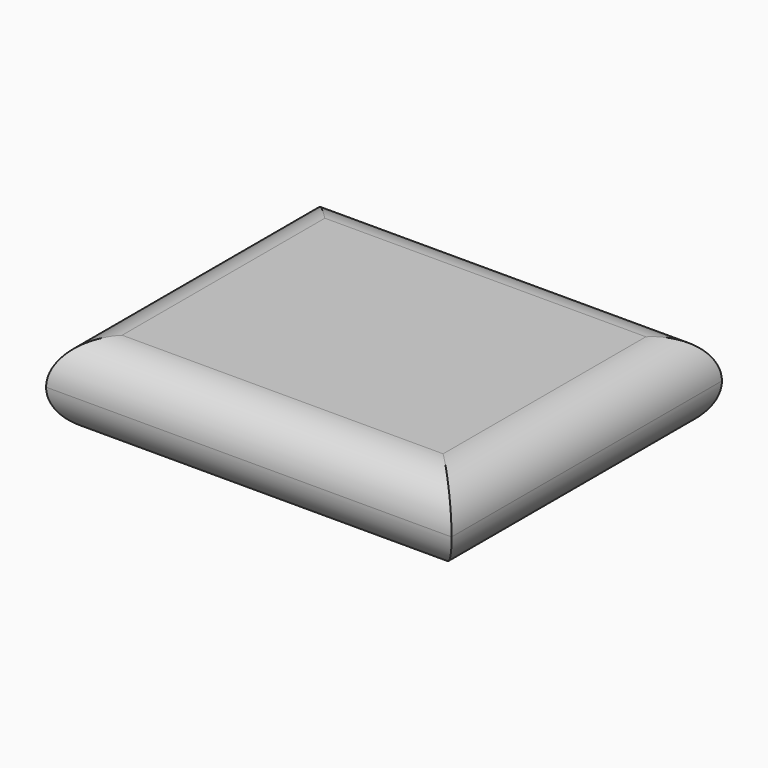
from build123d import *

# Parameters (mm, degrees)
F0_W     = 304.8
F0_H     = 254
F1_DEPTH = 63.5
F2_R     = 31.75
F3_R     = 31.74999


# Not quite as in the source:
# - a fillet or chamfer is up to 0.001 mm smaller than in the source, because OpenCascade refuses the exact size


with BuildPart() as f1:
    # F0 (on Top) → F1 (new body)
    with BuildSketch(Plane.XY):
        Rectangle(F0_W, F0_H)
    extrude(amount=F1_DEPTH)

    # F2
    f2_edges = [f1.edges().sort_by_distance(p)[0] for p in [
        (152.4, 0, 63.5),
        (0, 127, 63.5),
        (-152.4, 0, 63.5),
        (0, -127, 63.5),
    ]]
    fillet(f2_edges, radius=F2_R)

    # F3 (radius 31.75 in the source; OpenCascade refuses exactly that, so slightly less here)
    f3_edges = [f1.edges().sort_by_distance(p)[0] for p in [
        (152.4, 0, 0),
        (0, 127, 0),
        (-152.4, 0, 0),
        (0, -127, 0),
    ]]
    fillet(f3_edges, radius=F3_R)


solid = f1.part
